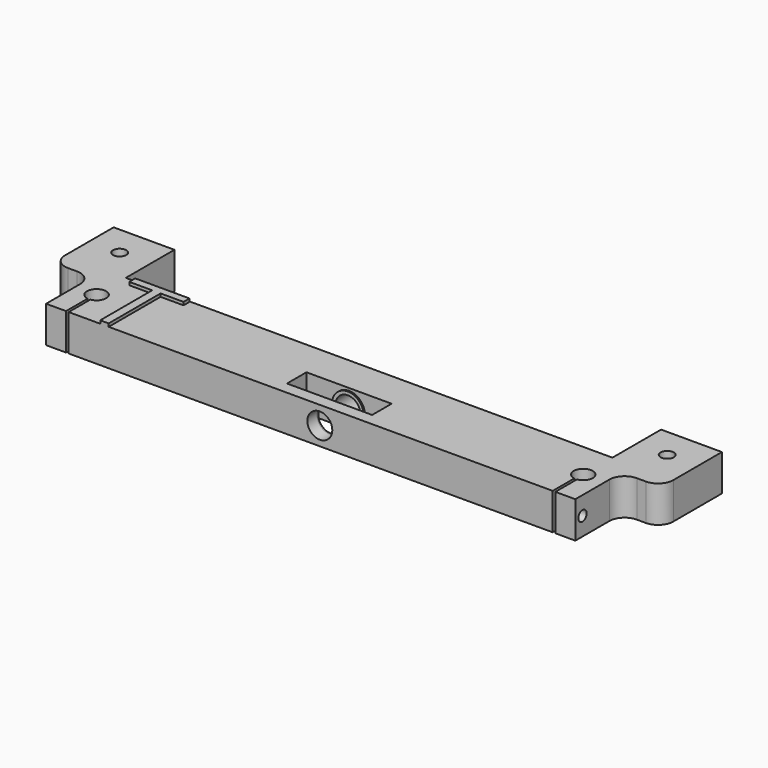
from build123d import *
from build123d import SkipClean  # not in build123d's __all__

# Parameters (mm, degrees)
F1_DEPTH      = 12
F3_DEPTH      = 12.001
F4_R          = 4.1
F5_DEPTH      = 20
F6_W          = 14
F6_H          = 8
F7_DEPTH      = 12.001
F8_R          = 5.1951476321
F8_R_2        = 4.1
F9_DEPTH      = 0.5
F10_R         = 5.2529872518
F10_R_2       = 4.1
F11_DEPTH     = 0.5
F12_TEXT_SIZE = 33.3333333333
F13_DEPTH     = 1
F14_R         = 1.4
F15_DEPTH     = 18
F14_R_2       = 1.7
F16_DEPTH     = 6.5630027184
F17_R         = 5
F18_R         = 1.4
F19_DEPTH     = 18
F18_R_2       = 1.7
F20_DEPTH     = 6.5630027184
F21_R         = 5
F22_W         = 20
F22_H         = 12
F23_DEPTH     = 20
F24_R         = 5
F26_R         = 2.175
F27_DEPTH     = 13.001


# Not quite as in the source:
# - after a boolean that leaves OpenCascade's solid faulty, fix() repairs it
# - Text() gives the source's letters only with a copy of the font that has no kerning and outlines rounded to 1/6400 em; it was checked with that copy


with BuildPart() as f1:
    # F0 (on Top) → F1 (new body)
    with BuildSketch(Plane.XY):
        Polygon((153.6500561982, 12.3083528318), (-46.3499438018, 12.3083528318), (-46.3499438018, 7.3083528318), (-33.3499438018, 7.3083528318), (-33.3499438018, -11.6916471682), (140.6500561982, -11.6916471682), (140.6500561982, 7.3083528318), (153.6500561982, 7.3083528318), align=None)
    extrude(amount=F1_DEPTH)

    # F2 (on face) → F3 (cut, through all)
    with BuildSketch(Plane.XY.offset(12)):
        with BuildLine():
            ThreePointArc((-25.9119465202, -2.8110474922), (-23.972740462, -1.758384762), (-23.1999438018, 0.3083528318))
            ThreePointArc((-23.1999438018, 0.3083528318), (-28.4166813955, 2.6855561715), (-26.7879410833, -2.8110474922))
            Line((-26.7879410833, -2.8110474922), (-26.7879410833, -2.4328390658))
            Line((-26.7879410833, -2.4328390658), (-25.9119465202, -2.4328390658))
            Line((-25.9119465202, -2.4328390658), (-25.9119465202, -2.8110474922))
        make_face()
        with BuildLine():
            Line((-26.7879410833, -2.4328390658), (-26.7879410833, -2.8110474922))
            ThreePointArc((-26.7879410833, -2.8110474922), (-26.3499438018, -2.8416471682), (-25.9119465202, -2.8110474922))
            Line((-25.9119465202, -2.8110474922), (-25.9119465202, -2.4328390658))
            Line((-25.9119465202, -2.4328390658), (-26.7879410833, -2.4328390658))
        make_face()
        with BuildLine():
            ThreePointArc((-25.9119465202, -2.8110474922), (-26.3499438018, -2.8416471682), (-26.7879410833, -2.8110474922))
            Line((-26.7879410833, -2.8110474922), (-26.7879410833, -11.6916471682))
            Line((-26.7879410833, -11.6916471682), (-25.9119465202, -11.6916471682))
            Line((-25.9119465202, -11.6916471682), (-25.9119465202, -2.8110474922))
        make_face()
        with BuildLine():
            ThreePointArc((134.0880534798, -2.8110474922), (136.027259538, -1.758384762), (136.8000561982, 0.3083528318))
            ThreePointArc((136.8000561982, 0.3083528318), (131.5833186045, 2.6855561715), (133.2120589167, -2.8110474922))
            Line((133.2120589167, -2.8110474922), (133.2120589167, -2.4328390658))
            Line((133.2120589167, -2.4328390658), (134.0880534798, -2.4328390658))
            Line((134.0880534798, -2.4328390658), (134.0880534798, -2.8110474922))
        make_face()
        with BuildLine():
            Line((133.2120589167, -2.4328390658), (133.2120589167, -2.8110474922))
            ThreePointArc((133.2120589167, -2.8110474922), (133.6500561982, -2.8416471682), (134.0880534798, -2.8110474922))
            Line((134.0880534798, -2.8110474922), (134.0880534798, -2.4328390658))
            Line((134.0880534798, -2.4328390658), (133.2120589167, -2.4328390658))
        make_face()
        with BuildLine():
            ThreePointArc((134.0880534798, -2.8110474922), (133.6500561982, -2.8416471682), (133.2120589167, -2.8110474922))
            Line((133.2120589167, -2.8110474922), (133.2120589167, -11.6916471682))
            Line((133.2120589167, -11.6916471682), (134.0880534798, -11.6916471682))
            Line((134.0880534798, -11.6916471682), (134.0880534798, -2.8110474922))
        make_face()
    extrude(amount=-F3_DEPTH, mode=Mode.SUBTRACT)

    # F4 (on face) → F5 (cut)
    with BuildSketch(Plane.XZ.offset(11.6916471682)):
        with Locations((56.6500561982, 6)):
            Circle(F4_R)
    extrude(amount=-F5_DEPTH, mode=Mode.SUBTRACT)

    # F6 (on face) → F7 (cut, through all)
    with BuildSketch(Plane.XY.offset(12)):
        with Locations((49.6500561982, -3.6916471682)):
            Rectangle(F6_W, F6_H)
        with Locations((63.6500561982, -3.6916471682)):
            Rectangle(F6_W, F6_H)
    extrude(amount=-F7_DEPTH, mode=Mode.SUBTRACT)

    # F8 (on face) → F9 (join)
    with BuildSketch(Plane.XZ.offset(-0.3083528318)):
        with Locations((56.6500561982, 6)):
            Circle(F8_R)
        with Locations((56.6500561982, 6)):
            Circle(F8_R_2, mode=Mode.SUBTRACT)
    extrude(amount=F9_DEPTH)

    # F10 (on face) → F11 (join)
    with BuildSketch(Plane(origin=(0, -7.6916471682, 0), x_dir=(-1, 0, 0), z_dir=(0, 1, 0))):
        with Locations((-56.6500561982, 6)):
            Circle(F10_R)
        with Locations((-56.6500561982, 6)):
            Circle(F10_R_2, mode=Mode.SUBTRACT)
    with SkipClean():  # cleaning this boolean's faces spoils the solid; the shape is the same uncleaned
        extrude(amount=F11_DEPTH)

    # F12 (on face) → F13 (join)
    with BuildSketch(Plane.XY.offset(12)):
        with Locations((-23.367214418, -11.6916471682)):
            Text('T', F12_TEXT_SIZE, font='Open Sans', text_align=(TextAlign.LEFT, TextAlign.BOTTOM))
    extrude(amount=F13_DEPTH)

    add(f1.part.fix(), mode=Mode.REPLACE)

    # F14 (on face) → F15 (cut)
    with BuildSketch(Plane.YZ.offset(140.6500561982)):
        with Locations((-8.7363375351, 6)):
            Circle(F14_R)
    extrude(amount=-F15_DEPTH, mode=Mode.SUBTRACT)

    # F14 (on face) → F16 (cut, through all)
    with BuildSketch(Plane.YZ.offset(140.6500561982)):
        with Locations((-8.7363375351, 6)):
            Circle(F14_R_2)
        with Locations((-8.7363375351, 6)):
            Circle(F14_R, mode=Mode.SUBTRACT)
        with Locations((-8.7363375351, 6)):
            Circle(F14_R)
    extrude(amount=-F16_DEPTH, mode=Mode.SUBTRACT)

    # F17
    f17_edges = [f1.edges().sort_by_distance(p)[0] for p in [
        (140.650056, 7.308353, 6),
    ]]
    fillet(f17_edges, radius=F17_R)

    # F18 (on face) → F19 (cut)
    with BuildSketch(Plane(origin=(-33.3499438018, 0, 0), x_dir=(0, -1, 0), z_dir=(-1, 0, 0))):
        with Locations((8.7602175772, 6.004051771)):
            Circle(F18_R)
    extrude(amount=-F19_DEPTH, mode=Mode.SUBTRACT)

    # F18 (on face) → F20 (cut, through all)
    with BuildSketch(Plane(origin=(-33.3499438018, 0, 0), x_dir=(0, -1, 0), z_dir=(-1, 0, 0))):
        with Locations((8.7602175772, 6.004051771)):
            Circle(F18_R_2)
        with Locations((8.7602175772, 6.004051771)):
            Circle(F18_R, mode=Mode.SUBTRACT)
        with Locations((8.7602175772, 6.004051771)):
            Circle(F18_R)
    extrude(amount=-F20_DEPTH, mode=Mode.SUBTRACT)

    # F21
    f21_edges = [f1.edges().sort_by_distance(p)[0] for p in [
        (-33.349944, 7.308353, 6),
    ]]
    fillet(f21_edges, radius=F21_R)

    # F22 (on face) → F23 (join)
    with BuildSketch(Plane(origin=(0, 12.3083528318, 0), x_dir=(-1, 0, 0), z_dir=(0, 1, 0))):
        with Locations((-143.6500561982, 6)):
            Rectangle(F22_W, F22_H)
        with Locations((36.3499438018, 6)):
            Rectangle(F22_W, F22_H)
    extrude(amount=F23_DEPTH)

    # F24
    f24_edges = [f1.edges().sort_by_distance(p)[0] for p in [
        (153.650056, 7.308353, 6),
        (-46.349944, 7.308353, 6),
    ]]
    fillet(f24_edges, radius=F24_R)

    # F26 (on face) → F27 (cut, through all)
    with BuildSketch(Plane(origin=(0, 0, 0), x_dir=(1, 0, 0), z_dir=(0, 0, -1))):
        with Locations((-36.3499438018, -22.3083528318)):
            Circle(F26_R)
        with Locations((143.6500561982, -22.3083528318)):
            Circle(F26_R)
    extrude(amount=-F27_DEPTH, mode=Mode.SUBTRACT)


solid = f1.part
